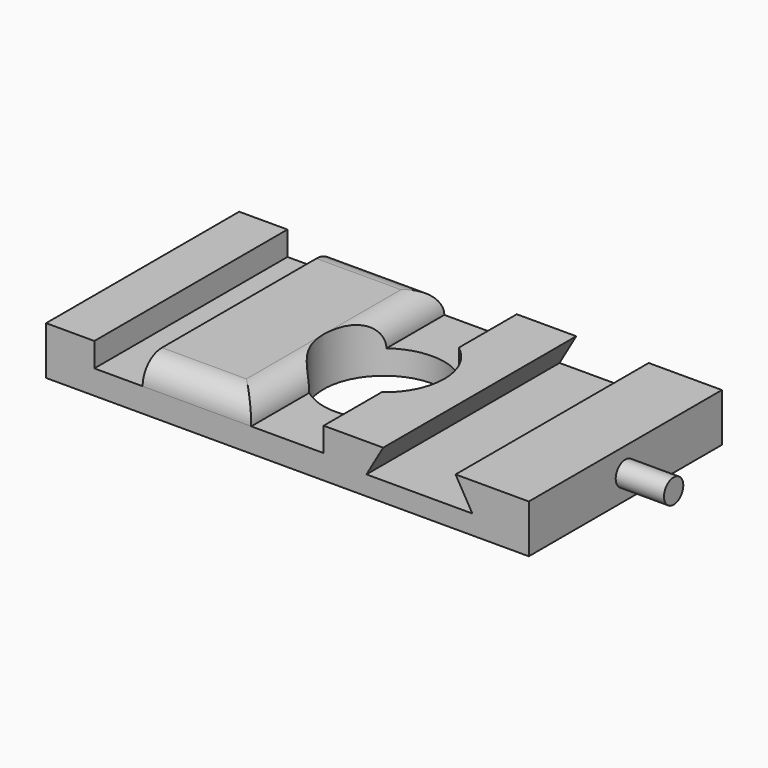
from build123d import *

# Parameters (mm, degrees)
F0_W     = 100
F0_H     = 50
F0_R     = 12.5
F1_DEPTH = 10
F2_W     = 10
F2_H     = 50
F3_DEPTH = 5
F5_DEPTH = 50.001
F6_R     = 2.5
F7_DEPTH = 10
F8_R     = 4.99999


# Not quite as in the source:
# - a fillet or chamfer is up to 0.001 mm smaller than in the source, because OpenCascade refuses the exact size


with BuildPart() as f1:
    # F0 (on Top) → F1 (new body)
    with BuildSketch(Plane.XY):
        Rectangle(F0_W, F0_H)
        Circle(F0_R, mode=Mode.SUBTRACT)
    extrude(amount=F1_DEPTH)

    # F2 (on face) → F3 (cut)
    with BuildSketch(Plane.XY.offset(10)):
        with Locations((-35, 0)):
            Rectangle(F2_W, F2_H)
        with BuildLine():
            Line((-7.5, -10), (-7.5, -25))
            Line((-7.5, -25), (7.5, -25))
            Line((7.5, -25), (7.5, -10))
            ThreePointArc((7.5, -10), (0, -12.5), (-7.5, -10))
        make_face()
        with BuildLine():
            Line((7.5, 25), (-7.5, 25))
            Line((-7.5, 25), (-7.5, 10))
            ThreePointArc((-7.5, 10), (0, 12.5), (7.5, 10))
            Line((7.5, 10), (7.5, 25))
        make_face()
    extrude(amount=-F3_DEPTH, mode=Mode.SUBTRACT)

    # F4 (on face) → F5 (cut, through all)
    with BuildSketch(Plane.XZ.offset(25)):
        Polygon((34.8284628647, 10), (19.8284628647, 10), (16.3643612496, 4), (38.2925644799, 4), align=None)
    extrude(amount=-F5_DEPTH, mode=Mode.SUBTRACT)

    # F6 (on face) → F7 (join)
    with BuildSketch(Plane.YZ.offset(50)):
        with Locations((0, 5)):
            Circle(F6_R)
    extrude(amount=F7_DEPTH)

    # F8 (radius 5 in the source; OpenCascade refuses exactly that, so slightly less here)
    f8_edges = [f1.edges().sort_by_distance(p)[0] for p in [
        (-18.75, -25, 10),
        (-18.75, 25, 10),
        (-7.5, -17.5, 10),
        (-7.5, 17.5, 10),
    ]]
    fillet(f8_edges, radius=F8_R)


solid = f1.part
